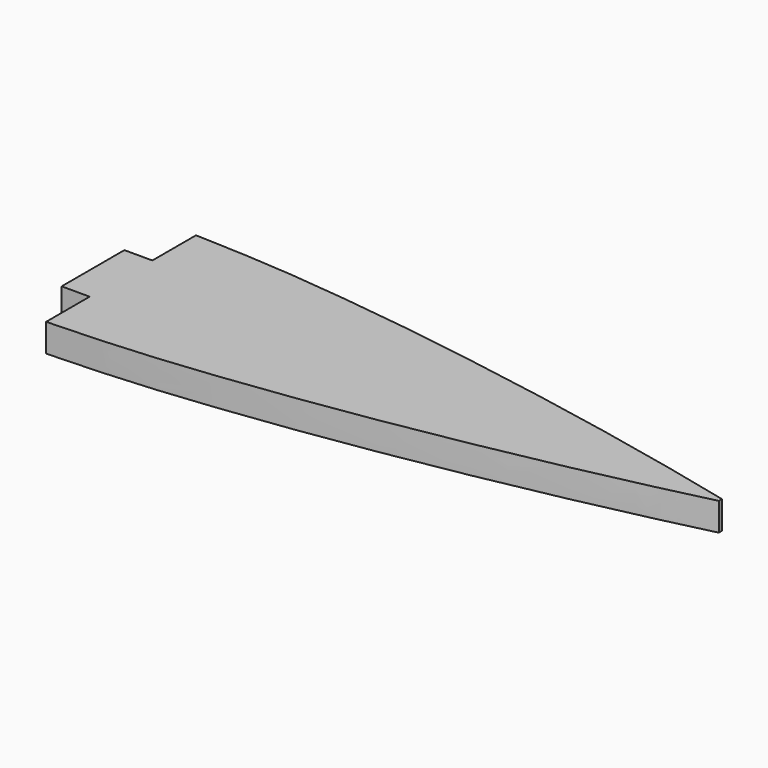
from build123d import *

# Parameters (mm, degrees)
F1_DEPTH = 3.175


with BuildPart() as f1:
    # F0 (on Top) → F1 (new body)
    with BuildSketch(Plane.XY):
        with BuildLine():
            Line((101.6, -0.224536), (101.6, 0.224536))
            add(Edge.make_bspline(
                [(101.6, 0.224536), (96.52, 1.434592), (97.928151728, 1.1118290006), (90.7318181321, 2.7613033932), (81.2086848949, 4.7190014757), (71.1474182421, 6.548791401), (60.9840942626, 8.1627459667), (50.7392971205, 9.4738409458), (42.0355898066, 10.3075715865), (35.8574731401, 10.5621488671), (33.655, 10.6191598962)],
                knots=[0, 0, 0, 0, 0.0277729611, 0.0555038819, 0.0946460349, 0.133701981, 0.1726784354, 0.211574615, 0.2503899882, 0.2759080683, 0.2759080683, 0.2759080683, 0.2759080683], degree=3))
            Line((33.655, 10.6191598962), (33.655, 4.445))
            Line((33.655, 4.445), (30.48, 4.445))
            Line((30.48, 4.445), (30.48, -4.445))
            Line((30.48, -4.445), (33.655, -4.445))
            Line((33.655, -4.445), (33.655, -10.6191598962))
            add(Edge.make_bspline(
                [(33.655, -10.6191598962), (35.8574731401, -10.5621488671), (42.0355898066, -10.3075715865), (50.7392971205, -9.4738409458), (60.9840942626, -8.1627459667), (71.1474182421, -6.548791401), (81.2086848949, -4.7190014757), (90.7318181321, -2.7613033932), (97.928151728, -1.1118290006), (96.52, -1.434592), (101.6, -0.224536)],
                knots=[0.7240919317, 0.7240919317, 0.7240919317, 0.7240919317, 0.7496100118, 0.788425385, 0.8273215646, 0.866298019, 0.9053539651, 0.9444961181, 0.9722270389, 1, 1, 1, 1], degree=3))
        make_face()
    extrude(amount=F1_DEPTH)


solid = f1.part
